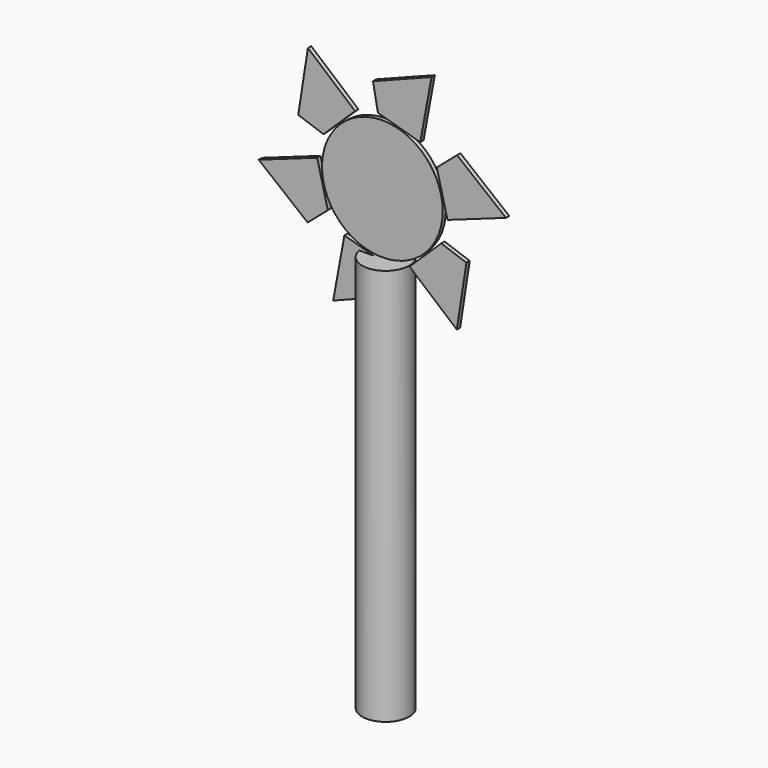
from build123d import *

# Parameters (mm, degrees)
F0_R     = 3.5714909455
F1_DEPTH = 60.452
F2_R     = 9.1876578043
F4_DEPTH = 0.635
F5_COUNT = 6


with BuildPart() as f1:
    # F0 (on Top) → F1 (new body)
    with BuildSketch(Plane.XY):
        Circle(F0_R)
    extrude(amount=F1_DEPTH)


with BuildPart() as f4:
    # F2 (on Front) → F4 (new body)
    with BuildSketch(Plane.XZ):
        with Locations((0, 69.8554515839)):
            Circle(F2_R)
    extrude(amount=F4_DEPTH)


with BuildPart() as f4b:
    # F2 (on Front) → F4, piece 2 (new body)
    with BuildSketch(Plane.XZ):
        Polygon((8.2955090329, 75.4171907902), (9.9212462083, 68.9142346382), (18.8200231642, 72.080142796), (11.3758547232, 78.0697092414), align=None)
    extrude(amount=F4_DEPTH)


with BuildPart() as f5_1:
    # F5: instance of F4b
    add(f4b.part.rotate(Axis((0, -0.635, 69.8554515839), (0, -1, 0)), 1 * 360 / F5_COUNT))


with BuildPart() as f5_2:
    # F5: instance of F4b
    add(f4b.part.rotate(Axis((0, -0.635, 69.8554515839), (0, -1, 0)), 2 * 360 / F5_COUNT))


with BuildPart() as f5_3:
    # F5: instance of F4b
    add(f4b.part.rotate(Axis((0, -0.635, 69.8554515839), (0, -1, 0)), 3 * 360 / F5_COUNT))


with BuildPart() as f5_4:
    # F5: instance of F4b
    add(f4b.part.rotate(Axis((0, -0.635, 69.8554515839), (0, -1, 0)), 4 * 360 / F5_COUNT))


with BuildPart() as f5_5:
    # F5: instance of F4b
    add(f4b.part.rotate(Axis((0, -0.635, 69.8554515839), (0, -1, 0)), 5 * 360 / F5_COUNT))


solid = Compound([f1.part, f4.part, f4b.part, f5_1.part, f5_2.part, f5_3.part, f5_4.part, f5_5.part])
